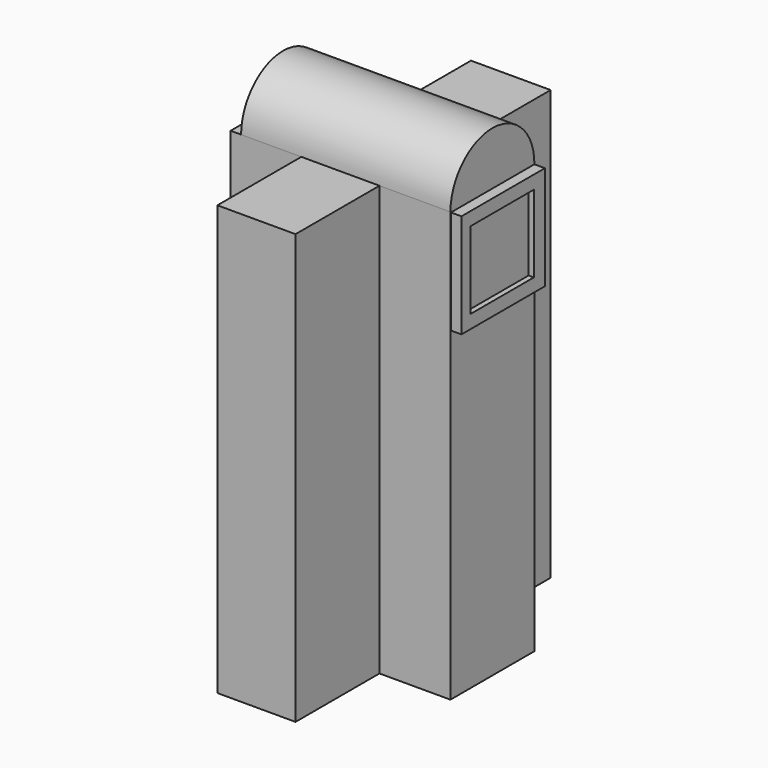
from build123d import *

# Parameters (mm, degrees)
F0_W      = 50.6787924096
F0_H      = 103.9609350264
F1_DEPTH  = 25.4
F4_W      = 18.917764537
F4_H      = 103.9609350264
F5_DEPTH  = 25.4
F6_W      = 19.2797044292
F6_H      = 103.9609350264
F7_DEPTH  = 25.4
F10_W     = 25.2526141703
F10_H     = 25.1658372581
F11_DEPTH = 2.54
F28_W     = 19.1976749338
F28_H     = 18.704187125
F29_DEPTH = 1.27
F30_W     = 19.0913220868
F30_H     = 18.744206056
F31_DEPTH = 1.27
F32_W     = 25.4
F32_H     = 25.8600655943
F32_W_2   = 19.0913220868
F32_H_2   = 18.744206056
F33_DEPTH = 2.54


# Not quite as in the source:
# - the program builds the solid bodies; features that only make, move or delete a surface that nothing else refers to are left out


with BuildPart() as f1:
    # F0 (on Front) → F1 (new body)
    with BuildSketch(Plane.XZ):
        with Locations((1.8223566003, -0.2603363246)):
            Rectangle(F0_W, F0_H)
    extrude(amount=F1_DEPTH)

    # F4 (on face) → F5 (join)
    with BuildSketch(Plane.XZ.offset(25.4)):
        with Locations((0.5206721835, -0.2603363246)):
            Rectangle(F4_W, F4_H)
    extrude(amount=F5_DEPTH)

    # F6 (on face) → F7 (join)
    with BuildSketch(Plane(origin=(0, 0, 0), x_dir=(-1, 0, 0), z_dir=(0, 1, 0))):
        with Locations((-1.1341772042, -0.2603363246)):
            Rectangle(F6_W, F6_H)
    extrude(amount=F7_DEPTH)

    # F9: sweep along a path in F8
    with BuildLine(Plane.XY.offset(51.7201311886)) as f9_path:
        Line((-23.5170396045, -12.7), (27.1617528051, -12.7))
    # F3 (on face) → F9 (sweep)
    with BuildSketch(Plane(origin=(-23.5170396045, 0, 0), x_dir=(0, -1, 0), z_dir=(-1, 0, 0))):
        with BuildLine():
            Line((0, 51.7201311886), (25.4, 51.7201311886))
            ThreePointArc((25.4, 51.7201311886), (12.7, 64.4201311886), (0, 51.7201311886))
        make_face()
    sweep(path=f9_path.line)

    # F10 (on face) → F11 (join)
    with BuildSketch(Plane.YZ.offset(27.1617528051)):
        with Locations((-12.6263070852, 38.9636550099)):
            Rectangle(F10_W, F10_H)
    extrude(amount=F11_DEPTH)

    # F28 (on face) → F29 (cut)
    with BuildSketch(Plane.YZ.offset(29.7017528051)):
        with Locations((-12.9288590979, 38.9715339988)):
            Rectangle(F28_W, F28_H)
    extrude(amount=-F29_DEPTH, mode=Mode.SUBTRACT)

    # F30 (on face) → F31 (cut)
    with BuildSketch(Plane(origin=(-23.5170396045, 0, 0), x_dir=(0, -1, 0), z_dir=(-1, 0, 0))):
        with Locations((12.9300323315, 38.8768771663)):
            Rectangle(F30_W, F30_H)
    extrude(amount=-F31_DEPTH, mode=Mode.SUBTRACT)

    # F32 (on face) → F33 (join)
    with BuildSketch(Plane(origin=(-23.5170396045, 0, 0), x_dir=(0, -1, 0), z_dir=(-1, 0, 0))):
        with Locations((12.7, 38.7900983915)):
            Rectangle(F32_W, F32_H)
        with Locations((12.9300323315, 38.8768771663)):
            Rectangle(F32_W_2, F32_H_2, mode=Mode.SUBTRACT)
    extrude(amount=F33_DEPTH)


solid = f1.part
